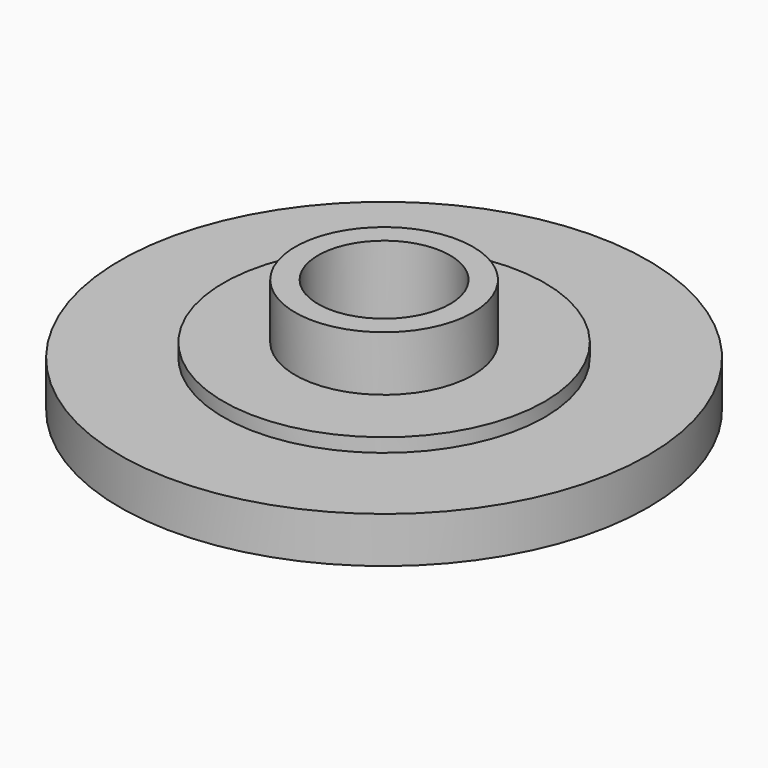
from build123d import *

# Parameters (mm, degrees)
F0_R     = 3.875
F1_DEPTH = 3
F0_R_2   = 7
F2_DEPTH = 0.6
F0_R_3   = 11.5
F3_DEPTH = 2
F4_DEPTH = 2
F6_T     = 1


# Not quite as in the source:
# - a shell that OpenCascade refuses in one call is made with other operations: the cavity is built on its own and cut out
# - the program builds the solid bodies; features that only make, move or delete a surface that nothing else refers to are left out


with BuildPart() as f1:
    # F0 (on Top) → F1 (new body)
    with BuildSketch(Plane.XY):
        Circle(F0_R)
    extrude(amount=F1_DEPTH)

    # F0 (on Top) → F2 (join)
    with BuildSketch(Plane.XY):
        Circle(F0_R_2)
        Circle(F0_R, mode=Mode.SUBTRACT)
    extrude(amount=F2_DEPTH)

    # F0 (on Top) → F3 (join)
    with BuildSketch(Plane.XY):
        Circle(F0_R_3)
        Circle(F0_R_2, mode=Mode.SUBTRACT)
        Circle(F0_R_2)
        Circle(F0_R, mode=Mode.SUBTRACT)
    extrude(amount=-F3_DEPTH)

    # F0 (on Top) → F4 (join)
    with BuildSketch(Plane.XY):
        Circle(F0_R)
    extrude(amount=-F4_DEPTH)

    # F6: shell of thickness 1, made by hand


with BuildPart() as f6_core1:
    # F6_t2: copy of F1
    add(f1.part)

    # the walls: a layer under each face that stays
    f6_faces = [f6_core1.faces().sort_by_distance(p)[0] for p in [
        (-3.875, 0, 1.8),
        (-4.6666666667, -4.6666666667, 0.6),
        (-7, 0, 0.3),
        (-7.6666666667, -7.6666666667, 0),
        (-11.5, 0, -1),
        (0, 0, -2),
    ]]
    thicken(f6_faces, amount=-F6_T, mode=Mode.SUBTRACT)

    # F6_s3 → F6_t4 (revolve, cut)
    with BuildSketch(Plane.XZ):
        Polygon((3.885, 0.61), (2.875, 0.6), (2.875, -0.4), (3.875, -0.4), align=None)
    revolve(axis=Axis((0, 0, 0.6), (0, 0, 1)), mode=Mode.SUBTRACT)

    # F6_s5 → F6_t6 (revolve, cut)
    with BuildSketch(Plane.XZ):
        Polygon((7.01, 0.01), (6, 0), (6, -1), (7, -1), align=None)
    revolve(axis=Axis((0, 0, 0), (0, 0, 1)), mode=Mode.SUBTRACT)


with BuildPart() as f1_1:
    add(f1.part)

    # what is left inside the walls is the cavity
    f6_cavity = [f6_core1.part.solids().sort_by_distance(p)[0] for p in [
        (0, -2, -0.99),
    ]]
    add(f6_cavity, mode=Mode.SUBTRACT)


solid = f1_1.part
